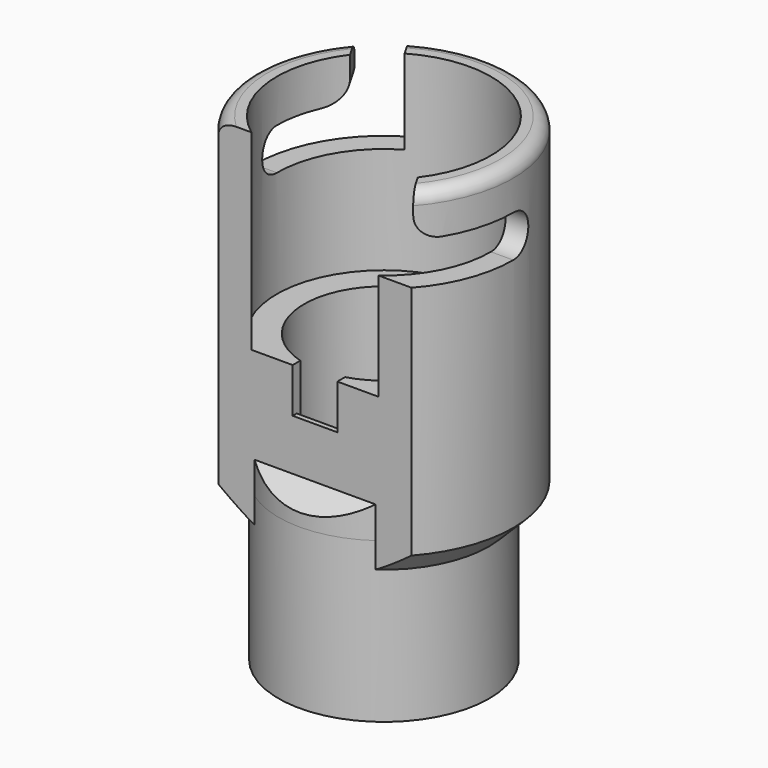
from build123d import *

# Parameters (mm, degrees)
F2_R          = 3.275
F3_DEPTH      = 25
F4_W          = 4
F4_H          = 6.55
F5_ANGLE      = 60
F6_W          = 4
F6_H          = 6.55
F7_ANGLE      = 60
F9_DEPTH      = 10
F10_W         = 32
F10_H         = 8
F11_DEPTH     = 50.0010001
F12_W         = 7
F12_H         = 7
F13_DEPTH     = 5
F15_DEPTH     = 3.5
F16_R         = 2
F17_R         = 3.4
F18_R         = 16.5
F18_R_2       = 12.5
F19_DEPTH     = 25
F20_T4_ANGLE  = 270.7214927844
F20_S5_R      = 20.275
F20_T6_DEPTH  = 31
F20_T11_ANGLE = 90.6289211612
F20_S12_R     = 20.275
F20_T13_DEPTH = 16
F21_T4_DEPTH  = 44.6904958407
F21_S5_R      = 16.5
F21_T6_DEPTH  = 24


# Not quite as in the source:
# - a fillet or chamfer that OpenCascade refuses, or shapes differently, is made with other operations: its cross-section is extruded or revolved along the edge and cut away or added


with BuildPart() as f1:
    # F0 (on Front) → F1 (revolve)
    with BuildSketch(Plane.XZ):
        Polygon((20.275, 50), (16.775, 50), (16.775, 20), (12.5, 20), (12.5, 0), (20.275, 0), align=None)
    revolve(axis=Axis((0, 0, 24.5366517103), (0, 0, 1)))

    # F2 (on Right) → F3 (cut, symmetric)
    with BuildSketch(Plane.YZ):
        with Locations((0, 40)):
            Circle(F2_R)
    extrude(amount=F3_DEPTH, both=True, mode=Mode.SUBTRACT)

    # F4 (on Front) → F5 (revolve, cut)
    with BuildSketch(Plane.XZ):
        with Locations((18.275, 40)):
            Rectangle(F4_W, F4_H)
    revolve(axis=Axis((0, 0, 25.1644738019), (0, 0, -1)), revolution_arc=F5_ANGLE, mode=Mode.SUBTRACT)

    # F6 (on Front) → F7 (revolve, cut)
    with BuildSketch(Plane.XZ):
        with Locations((-18.275, 40)):
            Rectangle(F6_W, F6_H)
    revolve(axis=Axis((0, 0, 23.5361852683), (0, 0, -1)), revolution_arc=F7_ANGLE, mode=Mode.SUBTRACT)

    # F8 (on face) → F9 (cut)
    with BuildSketch(Plane.XY.offset(50)):
        with BuildLine():
            Line((-8.3875, 14.5275761485), (-10.1375, 17.5586650617))
            ThreePointArc((-10.1375, 17.5586650617), (-12.8757169507, 15.6617859137), (-15.2663853672, 13.342155104))
            Line((-15.2663853672, 13.342155104), (-13.3941586478, 10.0993633026))
            ThreePointArc((-13.3941586478, 10.0993633026), (-11.1136146512, 12.5653569144), (-8.3875, 14.5275761485))
        make_face()
        with BuildLine():
            Line((8.3875, -14.5275761485), (10.1375, -17.5586650617))
            ThreePointArc((10.1375, -17.5586650617), (12.8757169507, -15.6617859137), (15.2663853672, -13.342155104))
            Line((15.2663853672, -13.342155104), (13.3941586478, -10.0993633026))
            ThreePointArc((13.3941586478, -10.0993633026), (11.1136146512, -12.5653569144), (8.3875, -14.5275761485))
        make_face()
    extrude(amount=-F9_DEPTH, mode=Mode.SUBTRACT)

    # F10 (on face) → F11 (cut, through all)
    with BuildSketch(Plane.XY.offset(50)):
        with Locations((0, -17.5)):
            Rectangle(F10_W, F10_H)
    extrude(amount=-F11_DEPTH, mode=Mode.SUBTRACT)

    # F12 (on face) → F13 (cut)
    with BuildSketch(Plane.XZ.offset(13.5)):
        with Locations((0, 16.5)):
            Rectangle(F12_W, F12_H)
    extrude(amount=-F13_DEPTH, mode=Mode.SUBTRACT)

    # F14 (on Right) → F15 (cut, symmetric)
    with BuildSketch(Plane.YZ):
        Polygon((-10.3, 13), (-12.7, 13), (-11.2893841543, 5), (-10.3, 5), align=None)
    extrude(amount=F15_DEPTH, both=True, mode=Mode.SUBTRACT)

    # F16
    f16_edges = [f1.edges().sort_by_distance(p)[0] for p in [
        (15.661786, 12.875717, 50),
        (-20.274727, -0.105295, 50),
    ]]
    fillet(f16_edges, radius=F16_R)

    # F17
    f17_edges = [f1.edges().sort_by_distance(p)[0] for p in [
        (-14.330272, 11.720759, 43.275),
        (14.330272, -11.720759, 43.275),
    ]]
    fillet(f17_edges, radius=F17_R)

    # F18 (on face) → F19 (join)
    with BuildSketch(Plane(origin=(0, 0, 0), x_dir=(1, 0, 0), z_dir=(0, 0, -1))):
        Circle(F18_R)
        Circle(F18_R_2, mode=Mode.SUBTRACT)
    extrude(amount=F19_DEPTH)

    # F20: chamfer of 4 on 2 edges, made by hand


with BuildPart() as f20_tool2:
    # F20_s3 → F20_t4 (revolve)
    with BuildSketch(Plane(origin=(0, 0, 0), x_dir=(0, 0, 1), z_dir=(0.9999207165, 0.0125920918, 0))):
        Polygon((0, 20.5), (-4, 16.5), (0, 16.5), align=None)
    revolve(axis=Axis((0, 0, 0), (0, 0, -1)), revolution_arc=F20_T4_ANGLE)

    # F20_s5 → F20_t6 (intersect, symmetric)
    with BuildSketch(Plane.XY.offset(-2)):
        Circle(F20_S5_R)
    extrude(amount=F20_T6_DEPTH, both=True, mode=Mode.INTERSECT)

    split(bisect_by=Plane.XZ.offset(13.5), keep=Keep.BOTTOM)


with BuildPart() as f1_1:
    add(f1.part)

    # F20_t1: union F20_tool2
    add(f20_tool2.part)


with BuildPart() as f20_tool9:
    # F20_s10 → F20_t11 (revolve)
    with BuildSketch(Plane.XZ):
        Polygon((20.5, 0), (16.5, -4), (16.5, 0), align=None)
    revolve(axis=Axis((0, 0, 0), (0, 0, -1)), revolution_arc=F20_T11_ANGLE)

    # F20_s12 → F20_t13 (intersect, symmetric)
    with BuildSketch(Plane.XY.offset(-2)):
        Circle(F20_S12_R)
    extrude(amount=F20_T13_DEPTH, both=True, mode=Mode.INTERSECT)

    split(bisect_by=Plane.XZ.offset(13.5), keep=Keep.BOTTOM)


with BuildPart() as f1_2:
    add(f1_1.part)

    # F20_t8: union F20_tool9
    add(f20_tool9.part)

    # F21: chamfer of 5 on 1 edges, made by hand


with BuildPart() as f21_tool2:
    # F21_s3 → F21_t4 (new body)
    with BuildSketch(Plane.YZ.offset(-22.3452479203)):
        Polygon((-18.5, 0), (-13.5, 5), (-13.5, 0), align=None)
    extrude(amount=F21_T4_DEPTH)

    # F21_s5 → F21_t6 (intersect, symmetric)
    with BuildSketch(Plane.XY.offset(2.5)):
        Circle(F21_S5_R)
    extrude(amount=F21_T6_DEPTH, both=True, mode=Mode.INTERSECT)


with BuildPart() as f1_3:
    add(f1_2.part)

    # F21_t1: union F21_tool2
    add(f21_tool2.part)


solid = f1_3.part
